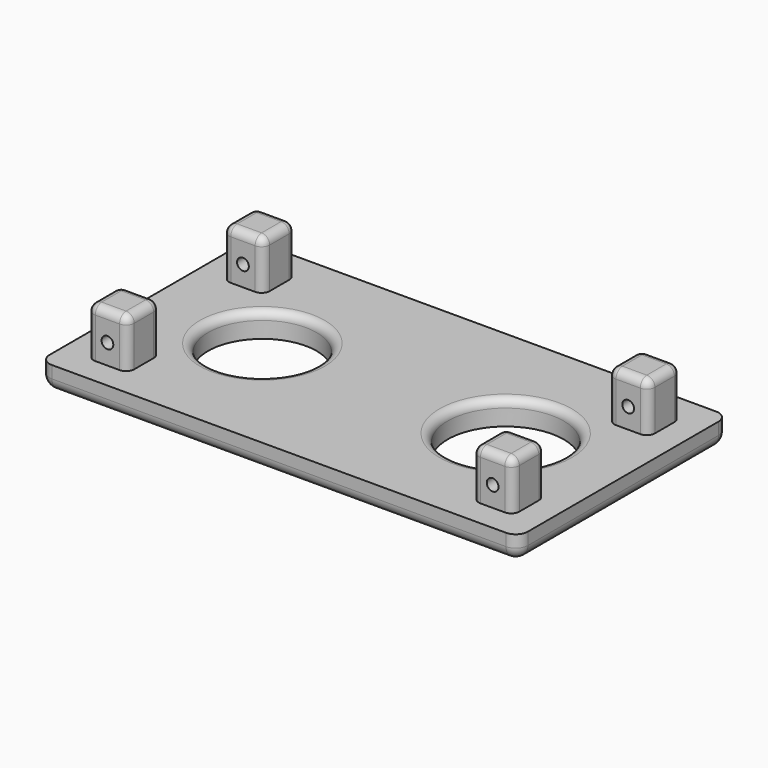
from build123d import *

# Parameters (mm, degrees)
F0_W         = 59.02
F0_H         = 32.4
F0_R         = 6.6906896399
F0_R_2       = 7.1640506352
F1_DEPTH     = 1.5
F2_W         = 5
F2_H         = 5
F3_DEPTH     = 6
F4_R         = 1
F5_R         = 1
F6_R         = 1.5
F7_T1_DEPTH  = 5.25
F7_S5_W      = 1.5
F7_S5_H      = 1.5
F7_T6_DEPTH  = 1.5
F7_S11_W     = 1.5
F7_S11_H     = 1.5
F7_T12_DEPTH = 1.5
F7_S17_W     = 1.5
F7_S17_H     = 1.5
F7_T18_DEPTH = 1.5
F7_S23_W     = 1.5
F7_S23_H     = 1.5
F7_T24_DEPTH = 1.5
F8_R         = 0.725
F9_DEPTH     = 35
F10_R        = 0.725
F11_DEPTH    = 35


# Not quite as in the source:
# - a fillet or chamfer that OpenCascade refuses, or shapes differently, is made with other operations: its cross-section is extruded or revolved along the edge and cut away or added


with BuildPart() as f1:
    # F0 (on Top) → F1 (new body, symmetric)
    with BuildSketch(Plane.XY):
        Rectangle(F0_W, F0_H)
        with Locations((-15.01, 0)):
            Circle(F0_R, mode=Mode.SUBTRACT)
        with Locations((15.01, 0)):
            Circle(F0_R_2, mode=Mode.SUBTRACT)
    extrude(amount=F1_DEPTH, both=True)

    # F2 (on face) → F3 (join)
    with BuildSketch(Plane.XY.offset(1.5)):
        with Locations((-23.76, -10.45)):
            Rectangle(F2_W, F2_H)
        with Locations((-23.76, 10.45)):
            Rectangle(F2_W, F2_H)
        with Locations((23.76, 10.45)):
            Rectangle(F2_W, F2_H)
        with Locations((23.76, -10.45)):
            Rectangle(F2_W, F2_H)
    extrude(amount=F3_DEPTH)

    # F4
    f4_edges = [f1.edges().sort_by_distance(p)[0] for p in [
        (26.26, -12.95, 4.5),
        (26.26, -7.95, 4.5),
        (26.26, 7.95, 4.5),
        (26.26, 12.95, 4.5),
        (21.26, -12.95, 4.5),
        (21.26, -7.95, 4.5),
        (-21.26, -12.95, 4.5),
        (-26.26, -12.95, 4.5),
        (-26.26, -7.95, 4.5),
        (-26.26, 7.95, 4.5),
        (-21.26, 7.95, 4.5),
        (21.26, 12.95, 4.5),
        (21.26, 7.95, 4.5),
        (-26.26, 12.95, 4.5),
        (-21.26, 12.95, 4.5),
        (-21.26, -7.95, 4.5),
    ]]
    fillet(f4_edges, radius=F4_R)

    # F5
    f5_edges = [f1.edges().sort_by_distance(p)[0] for p in [
        (-23.76, -7.95, 7.5),
        (-21.552893, -8.242893, 7.5),
        (-25.967107, -8.242893, 7.5),
        (-21.26, -10.45, 7.5),
        (-26.26, -10.45, 7.5),
        (-21.552893, -12.657107, 7.5),
        (-25.967107, -12.657107, 7.5),
        (-23.76, -12.95, 7.5),
        (-23.76, 12.95, 7.5),
        (-21.552893, 12.657107, 7.5),
        (-25.967107, 12.657107, 7.5),
        (-21.26, 10.45, 7.5),
        (-26.26, 10.45, 7.5),
        (-21.552893, 8.242893, 7.5),
        (-25.967107, 8.242893, 7.5),
        (-23.76, 7.95, 7.5),
        (23.76, 12.95, 7.5),
        (25.967107, 12.657107, 7.5),
        (21.552893, 12.657107, 7.5),
        (26.26, 10.45, 7.5),
        (21.26, 10.45, 7.5),
        (25.967107, 8.242893, 7.5),
        (21.552893, 8.242893, 7.5),
        (23.76, 7.95, 7.5),
        (23.76, -7.95, 7.5),
        (25.967107, -8.242893, 7.5),
        (21.552893, -8.242893, 7.5),
        (26.26, -10.45, 7.5),
        (21.26, -10.45, 7.5),
        (25.967107, -12.657107, 7.5),
        (21.552893, -12.657107, 7.5),
        (23.76, -12.95, 7.5),
        (7.845949, 0, 1.5),
        (-21.70069, 0, 1.5),
    ]]
    fillet(f5_edges, radius=F5_R)

    # F6
    f6_edges = [f1.edges().sort_by_distance(p)[0] for p in [
        (0, 16.2, -1.5),
        (-29.51, 0, -1.5),
        (0, -16.2, -1.5),
        (29.51, 0, -1.5),
    ]]
    fillet(f6_edges, radius=F6_R)

    # F7: fillet of radius 1.5 on 4 edges, made by hand

    # F7_s2 → F7_t1 (cut)
    with BuildSketch(Plane.XY):
        with BuildLine():
            ThreePointArc((29.51, 14.7), (29.0706601718, 15.7606601718), (28.01, 16.2))
            Line((28.01, 16.2), (29.51, 16.2))
            Line((29.51, 16.2), (29.51, 14.7))
        make_face()
        with BuildLine():
            ThreePointArc((-29.51, 14.7), (-29.0706601718, 15.7606601718), (-28.01, 16.2))
            Line((-28.01, 16.2), (-29.51, 16.2))
            Line((-29.51, 16.2), (-29.51, 14.7))
        make_face()
        with BuildLine():
            ThreePointArc((-28.01, -16.2), (-29.0706601718, -15.7606601718), (-29.51, -14.7))
            Line((-29.51, -14.7), (-29.51, -16.2))
            Line((-29.51, -16.2), (-28.01, -16.2))
        make_face()
        with BuildLine():
            ThreePointArc((28.01, -16.2), (29.0706601718, -15.7606601718), (29.51, -14.7))
            Line((29.51, -14.7), (29.51, -16.2))
            Line((29.51, -16.2), (28.01, -16.2))
        make_face()
    extrude(amount=F7_T1_DEPTH, mode=Mode.SUBTRACT)


with BuildPart() as f7_tool4:
    # F7_s5 → F7_t6 (new body)
    with BuildSketch(Plane.XZ.offset(14.7)):
        with Locations((28.76, -0.75)):
            Rectangle(F7_S5_W, F7_S5_H)
    extrude(amount=F7_T6_DEPTH)

    # F7_s7 → F7_t8 (revolve, cut)
    with BuildSketch(Plane(origin=(28.01, -14.7, 0), x_dir=(-0.7071067812, 0, 0.7071067812), z_dir=(0.7071067812, 0, 0.7071067812))):
        with BuildLine():
            ThreePointArc((0, -1.5), (1.5, 0), (0, 1.5))
            Line((0, 1.5), (0, -1.5))
        make_face()
    revolve(axis=Axis((28.01, -14.7, 0), (0, -1, 0)), mode=Mode.SUBTRACT)


with BuildPart() as f1_1:
    add(f1.part)

    # F7_t3: cut F7_tool4
    add(f7_tool4.part, mode=Mode.SUBTRACT)


with BuildPart() as f7_tool10:
    # F7_s11 → F7_t12 (new body)
    with BuildSketch(Plane.XZ.offset(14.7)):
        with Locations((-28.76, -0.75)):
            Rectangle(F7_S11_W, F7_S11_H)
    extrude(amount=F7_T12_DEPTH)

    # F7_s13 → F7_t14 (revolve, cut)
    with BuildSketch(Plane(origin=(-28.01, -14.7, 0), x_dir=(0.7071067812, 0, 0.7071067812), z_dir=(0.7071067812, 0, -0.7071067812))):
        with BuildLine():
            ThreePointArc((0, -1.5), (1.5, 0), (0, 1.5))
            Line((0, 1.5), (0, -1.5))
        make_face()
    revolve(axis=Axis((-28.01, -14.7, 0), (0, -1, 0)), mode=Mode.SUBTRACT)


with BuildPart() as f1_2:
    add(f1_1.part)

    # F7_t9: cut F7_tool10
    add(f7_tool10.part, mode=Mode.SUBTRACT)


with BuildPart() as f7_tool16:
    # F7_s17 → F7_t18 (new body)
    with BuildSketch(Plane.YZ.offset(-28.01)):
        with Locations((15.45, -0.75)):
            Rectangle(F7_S17_W, F7_S17_H)
    extrude(amount=-F7_T18_DEPTH)

    # F7_s19 → F7_t20 (revolve, cut)
    with BuildSketch(Plane(origin=(-28.01, 14.7, 0), x_dir=(0, -0.7071067812, 0.7071067812), z_dir=(0, -0.7071067812, -0.7071067812))):
        with BuildLine():
            ThreePointArc((0, -1.5), (1.5, 0), (0, 1.5))
            Line((0, 1.5), (0, -1.5))
        make_face()
    revolve(axis=Axis((-28.01, 14.7, 0), (-1, 0, 0)), mode=Mode.SUBTRACT)


with BuildPart() as f1_3:
    add(f1_2.part)

    # F7_t15: cut F7_tool16
    add(f7_tool16.part, mode=Mode.SUBTRACT)


with BuildPart() as f7_tool22:
    # F7_s23 → F7_t24 (new body)
    with BuildSketch(Plane.YZ.offset(28.01)):
        with Locations((15.45, -0.75)):
            Rectangle(F7_S23_W, F7_S23_H)
    extrude(amount=F7_T24_DEPTH)

    # F7_s25 → F7_t26 (revolve, cut)
    with BuildSketch(Plane(origin=(28.01, 14.7, 0), x_dir=(0, -0.7071067812, 0.7071067812), z_dir=(0, 0.7071067812, 0.7071067812))):
        with BuildLine():
            ThreePointArc((0, -1.5), (1.5, 0), (0, 1.5))
            Line((0, 1.5), (0, -1.5))
        make_face()
    revolve(axis=Axis((28.01, 14.7, 0), (1, 0, 0)), mode=Mode.SUBTRACT)


with BuildPart() as f1_4:
    add(f1_3.part)

    # F7_t21: cut F7_tool22
    add(f7_tool22.part, mode=Mode.SUBTRACT)

    # F8 (on face) → F9 (cut)
    with BuildSketch(Plane.XZ.offset(12.95)):
        with Locations((23.76, 4)):
            Circle(F8_R)
    extrude(amount=-F9_DEPTH, mode=Mode.SUBTRACT)

    # F10 (on face) → F11 (cut)
    with BuildSketch(Plane.XZ.offset(12.95)):
        with Locations((-23.76, 4)):
            Circle(F10_R)
    extrude(amount=-F11_DEPTH, mode=Mode.SUBTRACT)


solid = f1_4.part
